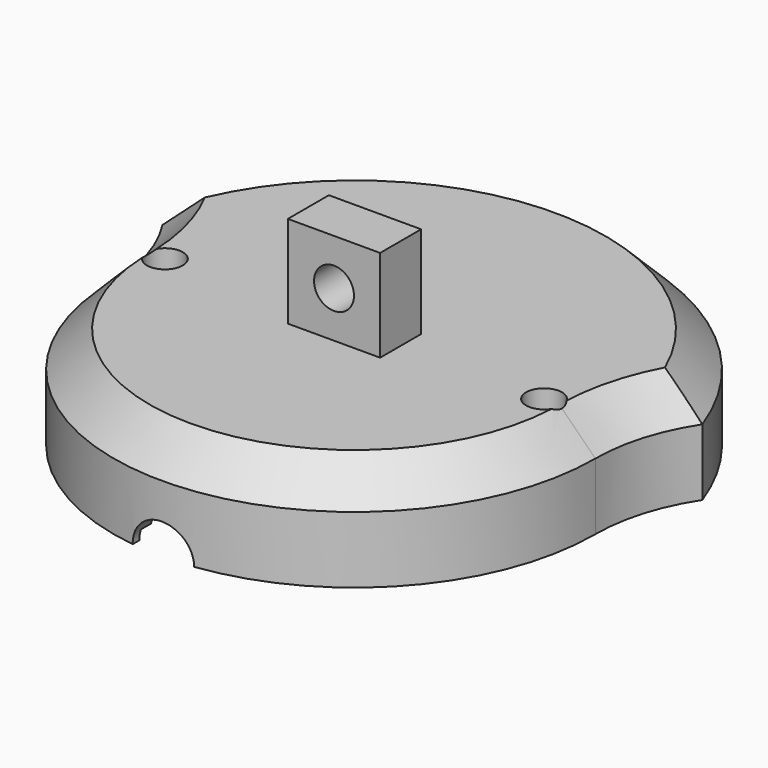
from build123d import *

# Parameters (mm, degrees)
F0_R         = 1
F1_DEPTH     = 5
F3_DEPTH     = 8
F5_DEPTH     = 1
F6_R         = 1
F7_DEPTH     = 7
F8_R         = 1.75
F9_DEPTH     = 8
F10_R        = 3
F11_DEPTH    = 23.501
F12_W        = 9
F12_H        = 9
F12_R        = 1.95
F13_DEPTH    = 2.5
F16_DEPTH    = 6.5
F17_DEPTH    = 7
F18_R        = 1.75
F19_DEPTH    = 28.001
F20_T2_ANGLE = 180
F20_T4_ANGLE = 63.0666087428
F20_T6_ANGLE = 177.2059132033
F20_T8_ANGLE = 63.0666087428


# Not quite as in the source:
# - a fillet or chamfer that OpenCascade refuses, or shapes differently, is made with other operations: its cross-section is extruded or revolved along the edge and cut away or added


with BuildPart() as f1:
    # F0 (on Top) → F1 (new body, symmetric)
    with BuildSketch(Plane.XY):
        with BuildLine():
            ThreePointArc((-26.3391343821, 9.5), (-24.2249616205, 4.9575872166), (-23.5, 0))
            ThreePointArc((-23.5, 0), (0, -23.5), (23.5, 0))
            ThreePointArc((23.5, 0), (24.2249616205, 4.9575872166), (26.3391343821, 9.5))
            ThreePointArc((26.3391343821, 9.5), (0, 28), (-26.3391343821, 9.5))
        make_face()
        with Locations((-18.5, 0)):
            Circle(F0_R, mode=Mode.SUBTRACT)
        with Locations((18.5, 0)):
            Circle(F0_R, mode=Mode.SUBTRACT)
    extrude(amount=F1_DEPTH, both=True)

    # F2 (on face) → F3 (cut)
    with BuildSketch(Plane(origin=(0, 0, -5), x_dir=(1, 0, 0), z_dir=(0, 0, -1))):
        with BuildLine():
            ThreePointArc((21.5, 0), (0, 21.5), (-21.5, 0))
            ThreePointArc((-21.5, 0), (-22.1675592341, -5.0230125511), (-24.12389255, -9.6973093298))
            ThreePointArc((-24.12389255, -9.6973093298), (0, -26), (24.12389255, -9.6973093298))
            ThreePointArc((24.12389255, -9.6973093298), (22.1675592341, -5.023012551), (21.5, 0))
        make_face()
    extrude(amount=-F3_DEPTH, mode=Mode.SUBTRACT)

    # F4 (on face) → F5 (cut)
    with BuildSketch(Plane(origin=(0, 0, -5), x_dir=(1, 0, 0), z_dir=(0, 0, -1))):
        with BuildLine():
            ThreePointArc((22.7, 0), (0, 22.7), (-22.7, 0))
            ThreePointArc((-22.7, 0), (-23.4028138558, -4.9851365308), (-25.4564681735, -9.5816610319))
            ThreePointArc((-25.4564681735, -9.5816610319), (0, -27.2), (25.4564681736, -9.5816610318))
            ThreePointArc((25.4564681736, -9.5816610318), (23.4028138558, -4.9851365307), (22.7, 0))
        make_face()
    extrude(amount=-F5_DEPTH, mode=Mode.SUBTRACT)

    # F6 (on face) → F7 (join, through all)
    with BuildSketch(Plane(origin=(0, 0, 3), x_dir=(1, 0, 0), z_dir=(0, 0, -1))):
        with BuildLine():
            ThreePointArc((-17.6723561014, -2.888314352), (-15.4992475751, 0.1511261164), (-17.9667347728, 2.9568534655))
            ThreePointArc((-17.9667347728, 2.9568534655), (-20.0762140714, 4.428973477), (-20.3324952956, 6.9885359735))
            ThreePointArc((-20.3324952956, 6.9885359735), (-22.8497447738, -0.1109553271), (-23.0826374703, -7.6399049653))
            ThreePointArc((-23.0826374703, -7.6399049653), (-20.9107637858, -4.6569183518), (-17.6723561014, -2.888314352))
        make_face()
        with Locations((-18.5, 0)):
            Circle(F6_R, mode=Mode.SUBTRACT)
        with BuildLine():
            ThreePointArc((20.3324952956, 6.9885359735), (20.0762140714, 4.428973477), (17.9667347728, 2.9568534655))
            ThreePointArc((17.9667347728, 2.9568534655), (15.4992475751, 0.1511261164), (17.6723561014, -2.888314352))
            ThreePointArc((17.6723561014, -2.888314352), (20.9107637858, -4.6569183518), (23.0826374703, -7.6399049653))
            ThreePointArc((23.0826374703, -7.6399049653), (22.9151781731, -0.0986538692), (20.3324952956, 6.9885359735))
        make_face()
        with Locations((18.5, 0)):
            Circle(F6_R, mode=Mode.SUBTRACT)
    extrude(amount=F7_DEPTH)

    # F8 (on face) → F9 (cut)
    with BuildSketch(Plane.XY.offset(5)):
        with Locations((-18.5, 0)):
            Circle(F8_R)
        with Locations((18.5, 0)):
            Circle(F8_R)
    extrude(amount=-F9_DEPTH, mode=Mode.SUBTRACT)

    # F10 (on Front) → F11 (cut, through all)
    with BuildSketch(Plane.XZ):
        with Locations((0, -5)):
            Circle(F10_R)
    extrude(amount=F11_DEPTH, mode=Mode.SUBTRACT)

    # F12 (on Front) → F13 (join, symmetric)
    with BuildSketch(Plane.XZ):
        with Locations((0, 9.5)):
            Rectangle(F12_W, F12_H)
        with Locations((0, 9.5)):
            Circle(F12_R, mode=Mode.SUBTRACT)
    extrude(amount=F13_DEPTH, both=True)

    # F15 (on face) → F16 (join)
    with BuildSketch(Plane(origin=(0, 0, -4), x_dir=(1, 0, 0), z_dir=(0, 0, -1))):
        with BuildLine():
            ThreePointArc((10.5675868988, -20.9899048863), (0, -23.5), (-10.5675868988, -20.9899048863))
            ThreePointArc((-10.5675868988, -20.9899048863), (-13.6551032171, -20.8795666046), (-15.75, -23.1503239718))
            ThreePointArc((-15.75, -23.1503239718), (0, -28), (15.75, -23.1503239718))
            ThreePointArc((15.75, -23.1503239718), (13.6551032171, -20.8795666046), (10.5675868988, -20.9899048863))
        make_face()
    extrude(amount=F16_DEPTH)

    # F15 (on face) → F17 (join, through all)
    with BuildSketch(Plane(origin=(0, 0, -4), x_dir=(1, 0, 0), z_dir=(0, 0, -1))):
        with BuildLine():
            ThreePointArc((10.5675868988, -20.9899048863), (0, -23.5), (-10.5675868988, -20.9899048863))
            ThreePointArc((-10.5675868988, -20.9899048863), (-13.6551032171, -20.8795666046), (-15.75, -23.1503239718))
            ThreePointArc((-15.75, -23.1503239718), (0, -28), (15.75, -23.1503239718))
            ThreePointArc((15.75, -23.1503239718), (13.6551032171, -20.8795666046), (10.5675868988, -20.9899048863))
        make_face()
    extrude(amount=-F17_DEPTH)

    # F18 (on Front) → F19 (cut, through all)
    with BuildSketch(Plane.XZ):
        with Locations((0, -7.75)):
            Circle(F18_R)
    extrude(amount=-F19_DEPTH, mode=Mode.SUBTRACT)

    # F20: chamfer of 3.5 on 4 edges, made by hand

    # F20_s1 → F20_t2 (revolve, cut)
    with BuildSketch(Plane.XZ):
        Polygon((-20, 5), (-23.5, 1.5), (-23.5, 5), align=None)
    revolve(axis=Axis((0, 0, 5), (0, 0, 1)), revolution_arc=F20_T2_ANGLE, mode=Mode.SUBTRACT)

    # F20_s3 → F20_t4 (revolve, cut)
    with BuildSketch(Plane.XZ):
        Polygon((23.5, 1.5), (20, 5), (23.5, 5), align=None)
    revolve(axis=Axis((40.8134960885, 0, 5), (0, 0, -1)), revolution_arc=F20_T4_ANGLE, mode=Mode.SUBTRACT)

    # F20_s5 → F20_t6 (revolve, cut)
    with BuildSketch(Plane(origin=(0, 0, 0), x_dir=(0, 0, 1), z_dir=(0.0243805911, -0.9997027492, 0))):
        Polygon((1.5, -28), (5, -24.5), (5, -28), align=None)
    revolve(axis=Axis((0, 0, 5), (0, 0, 1)), revolution_arc=F20_T6_ANGLE, mode=Mode.SUBTRACT)

    # F20_s7 → F20_t8 (revolve, cut)
    with BuildSketch(Plane(origin=(-32.4398868868, 16.4814724869, 0), x_dir=(0, 0, 1), z_dir=(-0.8915337049, 0.4529543608, 0))):
        Polygon((5, 2.326845056), (1.5, -1.173154944), (5, -1.173154944), align=None)
    revolve(axis=Axis((-40.8134960885, 0, 5), (0, 0, -1)), revolution_arc=F20_T8_ANGLE, mode=Mode.SUBTRACT)


solid = f1.part
